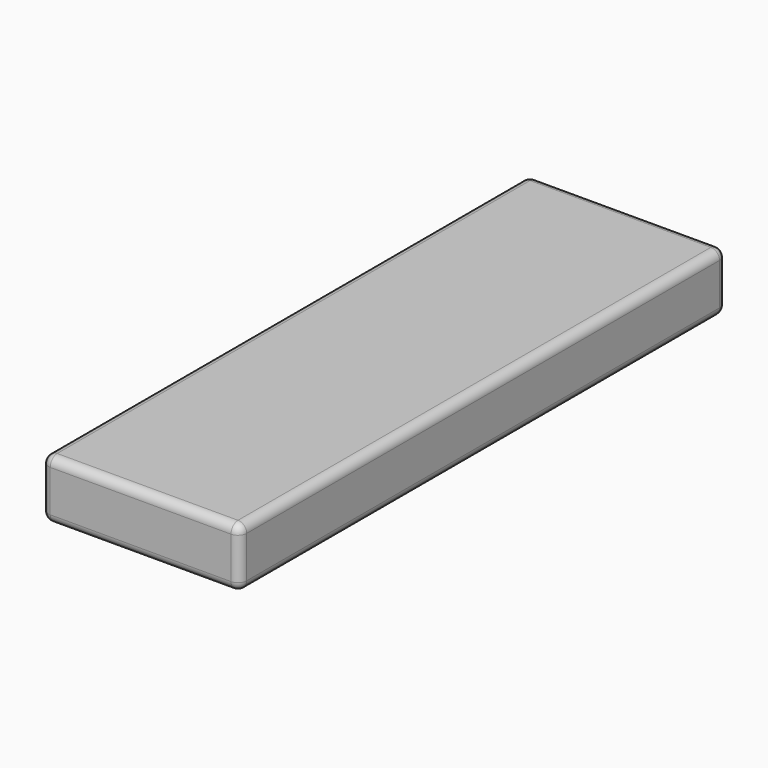
from build123d import *

# Parameters (mm, degrees)
F0_W     = 11.4
F0_H     = 3.4
F1_DEPTH = 35
F2_R     = 0.5


with BuildPart() as f1:
    # F0 (on Front) → F1 (new body)
    with BuildSketch(Plane.XZ):
        Rectangle(F0_W, F0_H)
    extrude(amount=F1_DEPTH)

    # F2
    f2_edges = [f1.edges().sort_by_distance(p)[0] for p in [
        (5.7, -35, 0),
        (0, -35, 1.7),
        (-5.7, -35, 0),
        (0, -35, -1.7),
        (5.7, -17.5, -1.7),
        (5.7, -17.5, 1.7),
        (5.7, 0, 0),
        (-5.7, -17.5, 1.7),
        (-5.7, -17.5, -1.7),
        (-5.7, 0, 0),
        (0, 0, 1.7),
        (0, 0, -1.7),
    ]]
    fillet(f2_edges, radius=F2_R)


solid = f1.part
